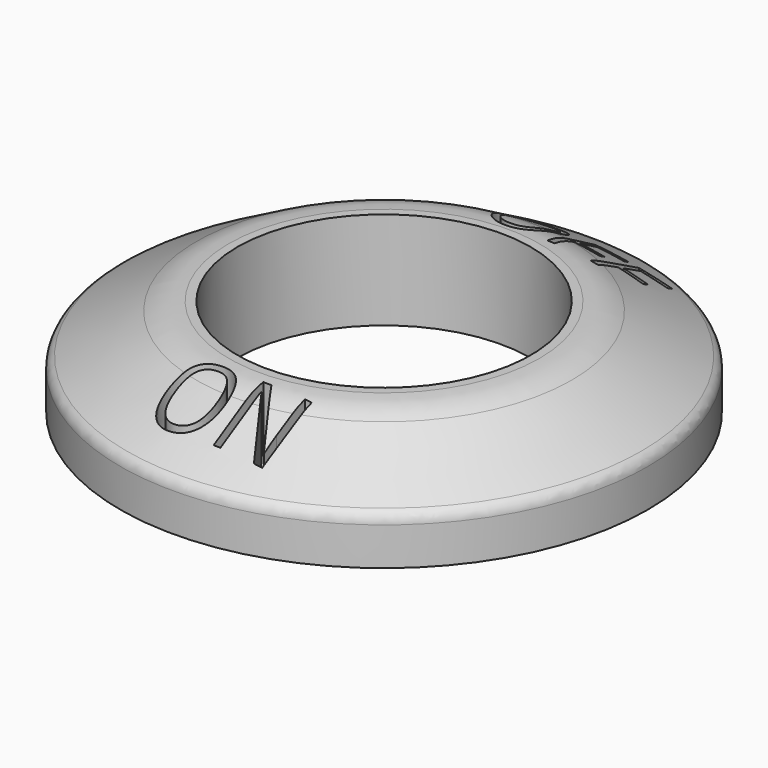
from build123d import *

# Parameters (mm, degrees)
F0_R           = 20.25
F3_DEPTH       = 3.5
F3_FACE_R      = 20.25
F2_R           = 13.25
F5_D           = 22.5
F5_DEPTH       = 30
F5_TIP         = 6.7596819641
F6_R           = 5
F7_R           = 1
F8_TEXT_SIZE   = 6.6694456023
F8_TEXT_SIZE_2 = 6.4662793635
F9_DEPTH       = 5


# Not quite as in the source:
# - Text() gives the source's letters only with a copy of the font that has no kerning and outlines rounded to 1/6400 em; it was checked with that copy


with BuildPart() as f3:
    # F0 (on Top) → F3 (new body)
    with BuildSketch(Plane.XY):
        Circle(F0_R)
    extrude(amount=F3_DEPTH)

    # F3_face (on face) → F4 section 0
    with BuildSketch(Plane.XY.offset(3.5)):
        Circle(F3_FACE_R)
    # F2 (on offset) → F4 section 1
    with BuildSketch(Plane.XY.offset(7.5)):
        Circle(F2_R)
    loft()

    # F5
    with Locations(Plane(origin=(0, 0, 0), x_dir=(1, 0, 0), z_dir=(0, 0, -1))):
        with Locations((0, 0)):
            Hole(F5_D / 2, depth=F5_DEPTH)
            with Locations((0, 0, -(F5_DEPTH + F5_TIP / 2))):  # 118° drill point
                Cone(0, F5_D / 2, F5_TIP, mode=Mode.SUBTRACT)

    # F6
    f6_edges = [f3.edges().sort_by_distance(p)[0] for p in [
        (-13.25, 0, 7.5),
    ]]
    fillet(f6_edges, radius=F6_R)

    # F7
    f7_edges = [f3.edges().sort_by_distance(p)[0] for p in [
        (-20.25, 0, 3.5),
    ]]
    fillet(f7_edges, radius=F7_R)

    # F8 (on offset) → F9 (cut)
    with BuildSketch(Plane.XY.offset(7.5)):
        with Locations((-5, -17.4008111387)):
            Text('ON', F8_TEXT_SIZE, font='Open Sans', text_align=(TextAlign.LEFT, TextAlign.BOTTOM))
        with Locations((-3.0068586438, 12.3242985253)):
            Text('OFF', F8_TEXT_SIZE_2, font='Open Sans', text_align=(TextAlign.LEFT, TextAlign.BOTTOM))
    extrude(amount=-F9_DEPTH, mode=Mode.SUBTRACT)


solid = f3.part
